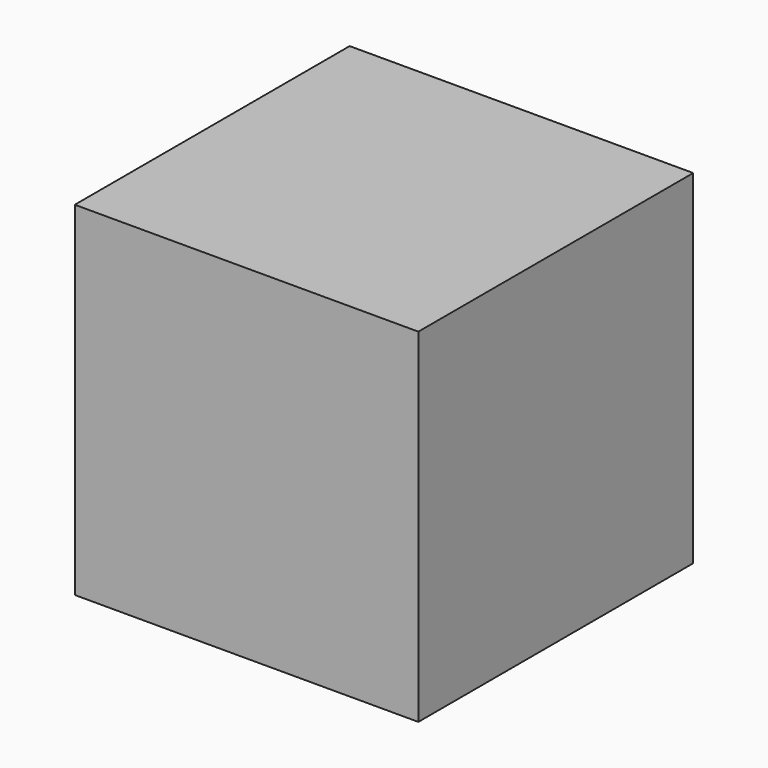
from build123d import *

# Parameters (mm, degrees)
F1_W     = 101.6
F1_H     = 101.6
F2_DEPTH = 50.8


# Not quite as in the source:
# - a variable given as a bare number and used for a length is read in inches; the dataset says mm whatever the document's units were


with BuildPart() as f2:
    # F1 (on Front) → F2 (new body, symmetric)
    with BuildSketch(Plane.XZ):
        with Locations((1.4030579478, -0.0212566953)):
            Rectangle(F1_W, F1_H)
    extrude(amount=F2_DEPTH, both=True)


solid = f2.part
